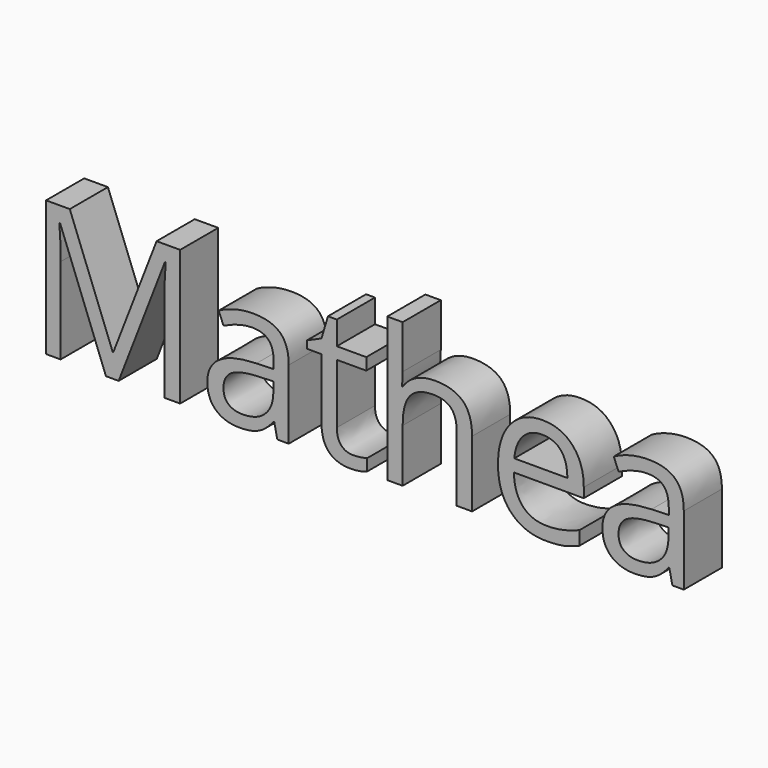
from build123d import *

# Parameters (mm, degrees)
F0_TEXT_SIZE = 101.037370041
F1_DEPTH     = 25.4


# Not quite as in the source:
# - Text() gives the source's letters only with a copy of the font that has no kerning and outlines rounded to 1/6400 em; it was checked with that copy


with BuildPart() as f1:
    # F0 (on Front) → F1 (new body)
    with BuildSketch(Plane.XZ):
        with Locations((-161.927412264, -18.2866863906)):
            Text('Mathea', F0_TEXT_SIZE, font='Open Sans', text_align=(TextAlign.LEFT, TextAlign.BOTTOM))
    extrude(amount=F1_DEPTH)


solid = f1.part
